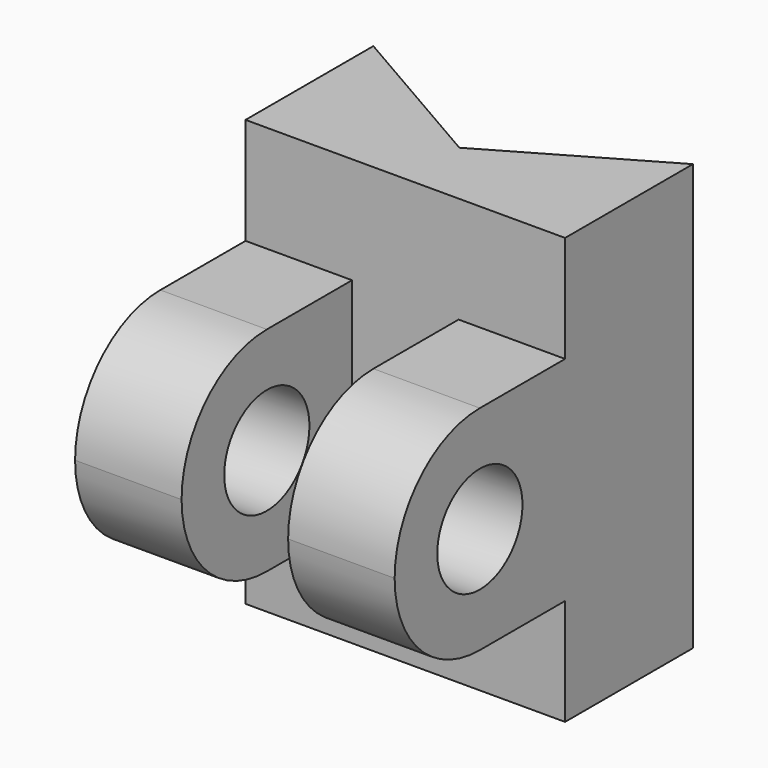
from build123d import *

# Parameters (mm, degrees)
F0_W     = 30
F0_H     = 40
F1_DEPTH = 15
F2_W     = 10
F2_H     = 20
F3_DEPTH = 20
F4_R     = 5
F5_DEPTH = 30.001
F6_R     = 9.99999
F8_DEPTH = 40.001


# Not quite as in the source:
# - a fillet or chamfer is up to 0.001 mm smaller than in the source, because OpenCascade refuses the exact size


with BuildPart() as f1:
    # F0 (on Front) → F1 (new body)
    with BuildSketch(Plane.XZ):
        Rectangle(F0_W, F0_H)
    extrude(amount=F1_DEPTH)

    # F2 (on face) → F3 (join)
    with BuildSketch(Plane.XZ.offset(15)):
        with Locations((-10, 0)):
            Rectangle(F2_W, F2_H)
        with Locations((10, 0)):
            Rectangle(F2_W, F2_H)
    extrude(amount=F3_DEPTH)

    # F4 (on face) → F5 (cut, through all)
    with BuildSketch(Plane.YZ.offset(15)):
        with Locations((-25, 0)):
            Circle(F4_R)
    extrude(amount=-F5_DEPTH, mode=Mode.SUBTRACT)

    # F6 (radius 10 in the source; OpenCascade refuses exactly that, so slightly less here)
    f6_edges = [f1.edges().sort_by_distance(p)[0] for p in [
        (10, -35, 10),
        (-10, -35, 10),
        (-10, -35, -10),
        (10, -35, -10),
    ]]
    fillet(f6_edges, radius=F6_R)

    # F7 (on face) → F8 (cut, through all)
    with BuildSketch(Plane.XY.offset(20)):
        Polygon((15, 0), (-15, 0), (0, -8.6602540378), align=None)
    extrude(amount=-F8_DEPTH, mode=Mode.SUBTRACT)


solid = f1.part
